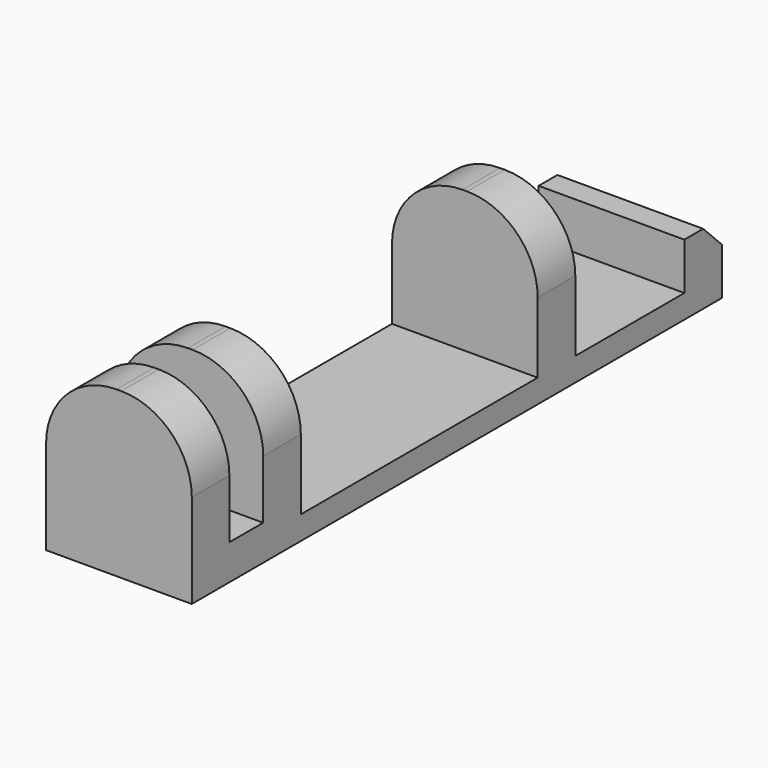
from build123d import *

# Parameters (mm, degrees)
F0_W     = 6.2
F0_H     = 2
F0_H_2   = 12.6
F0_H_3   = 1.8
F0_H_4   = 5.8
F1_DEPTH = 1
F2_DEPTH = 6
F3_R     = 3
F4_DEPTH = 0.5
F5_DEPTH = 2
F6_SIZE  = 1


with BuildPart() as f1:
    # F0 (on Top) → F1 (new body)
    with BuildSketch(Plane.XY):
        with Locations((0, 15.1)):
            Rectangle(F0_W, F0_H)
        with Locations((0, -11.1)):
            Rectangle(F0_W, F0_H)
        Rectangle(F0_W, F0_H_2)
        with Locations((0, -7.3)):
            Rectangle(F0_W, F0_H)
        with Locations((0, -9.2)):
            Rectangle(F0_W, F0_H_3)
        with Locations((0, 7.3)):
            Rectangle(F0_W, F0_H)
        with Locations((0, 11.2)):
            Rectangle(F0_W, F0_H_4)
    extrude(amount=-F1_DEPTH)

    # F0 (on Top) → F2 (join)
    with BuildSketch(Plane.XY):
        with Locations((0, 7.3)):
            Rectangle(F0_W, F0_H)
        with Locations((0, -7.3)):
            Rectangle(F0_W, F0_H)
        with Locations((0, -11.1)):
            Rectangle(F0_W, F0_H)
    extrude(amount=F2_DEPTH)

    # F3
    f3_edges = [f1.edges().sort_by_distance(p)[0] for p in [
        (-3.1, 7.3, 6),
        (-3.1, -7.3, 6),
        (-3.1, -11.1, 6),
        (3.1, 7.3, 6),
        (3.1, -7.3, 6),
        (3.1, -11.1, 6),
    ]]
    fillet(f3_edges, radius=F3_R)

    # F0 (on Top) → F4 (join)
    with BuildSketch(Plane.XY):
        with Locations((0, -9.2)):
            Rectangle(F0_W, F0_H_3)
    extrude(amount=F4_DEPTH)

    # F0 (on Top) → F5 (join)
    with BuildSketch(Plane.XY):
        with Locations((0, 15.1)):
            Rectangle(F0_W, F0_H)
    extrude(amount=F5_DEPTH)

    # F6
    f6_edges = [f1.edges().sort_by_distance(p)[0] for p in [
        (0, 16.1, 2),
    ]]
    chamfer(f6_edges, length=F6_SIZE)


solid = f1.part
